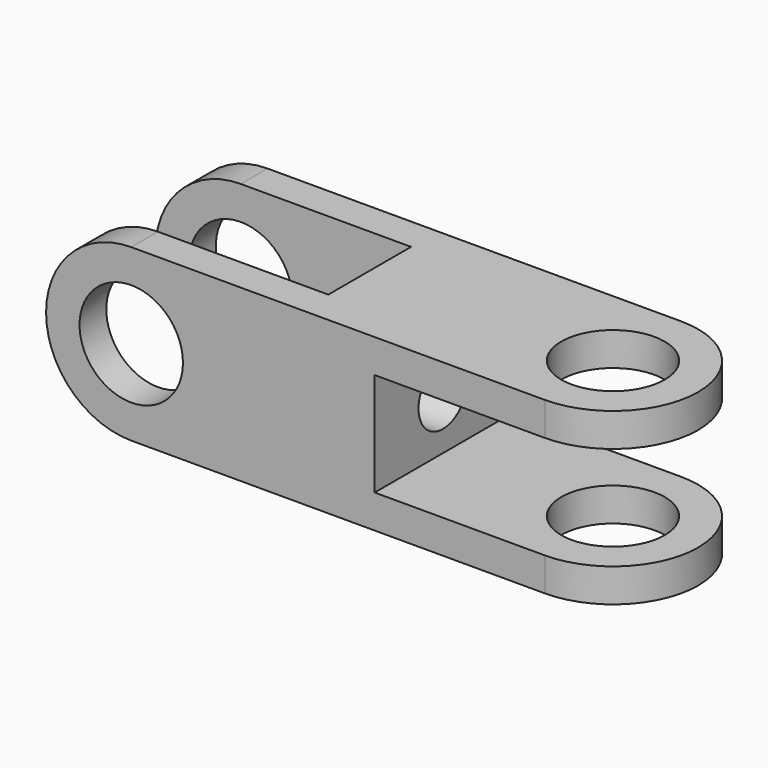
from build123d import *

# Parameters (mm, degrees)
F0_R     = 8.5
F1_DEPTH = 28
F2_R     = 8.5
F2_W     = 84
F2_H     = 17
F3_DEPTH = 28.001
F4_R     = 13.99999
F5_R     = 5
F6_DEPTH = 54.0266669521


# Not quite as in the source:
# - a fillet or chamfer is up to 0.001 mm smaller than in the source, because OpenCascade refuses the exact size


with BuildPart() as f1:
    # F0 (on Top) → F1 (new body)
    with BuildSketch(Plane.XY):
        with BuildLine():
            Line((41, 14), (-41, 14))
            Line((-41, 14), (-41, 8.5))
            Line((-41, 8.5), (1, 8.5))
            Line((1, 8.5), (1, -8.5))
            Line((1, -8.5), (-41, -8.5))
            Line((-41, -8.5), (-41, -14))
            Line((-41, -14), (41, -14))
            ThreePointArc((41, -14), (55, 0), (41, 14))
        make_face()
        with Locations((41, 0)):
            Circle(F0_R, mode=Mode.SUBTRACT)
    extrude(amount=F1_DEPTH)

    # F2 (on face) → F3 (cut, through all)
    with BuildSketch(Plane.XZ.offset(14)):
        with Locations((-27, 14)):
            Circle(F2_R)
        with Locations((55.0256669521, 14)):
            Rectangle(F2_W, F2_H)
    extrude(amount=-F3_DEPTH, mode=Mode.SUBTRACT)

    # F4 (radius 14 in the source; OpenCascade refuses exactly that, so slightly less here)
    f4_edges = [f1.edges().sort_by_distance(p)[0] for p in [
        (-41, 11.25, 28),
        (-41, 11.25, 0),
        (-41, -11.25, 28),
        (-41, -11.25, 0),
    ]]
    fillet(f4_edges, radius=F4_R)

    # F5 (on face) → F6 (cut, through all)
    with BuildSketch(Plane.YZ.offset(13.0256669521)):
        with Locations((0, 14)):
            Circle(F5_R)
    extrude(amount=-F6_DEPTH, mode=Mode.SUBTRACT)


solid = f1.part
